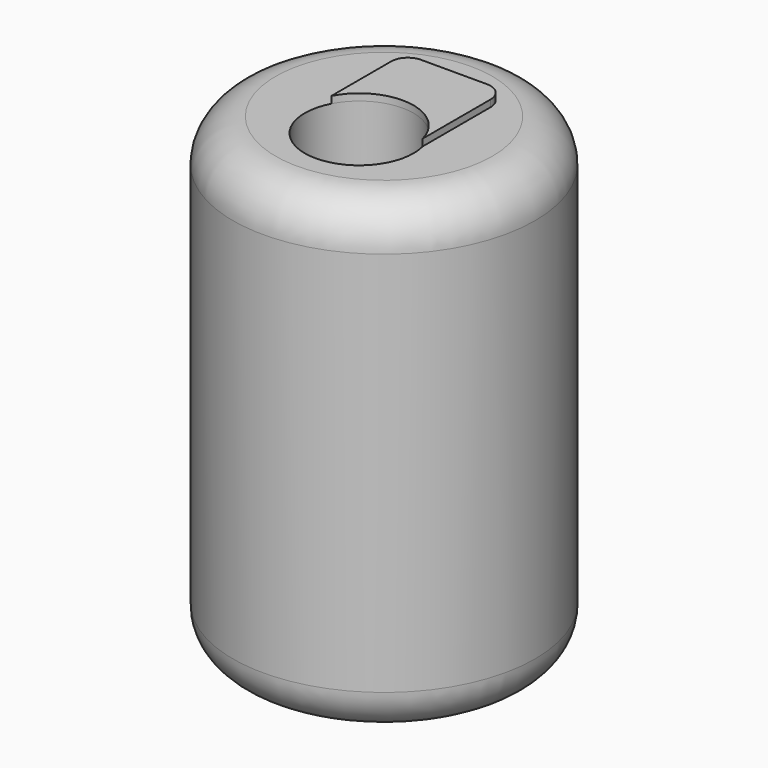
from build123d import *

# Parameters (mm, degrees)
F0_R     = 17.6630626633
F1_DEPTH = 55.1
F2_R     = 5
F3_R     = 6.360255015
F4_DEPTH = 4.4
F5_DEPTH = 9.1
F6_DEPTH = 6.2
F8_DEPTH = 0.8
F9_R     = 2.1727922061
F10_R    = 1.9313708499


# Not quite as in the source:
# - the program builds the solid bodies; features that only make, move or delete a surface that nothing else refers to are left out


with BuildPart() as f1:
    # F0 (on Top) → F1 (new body)
    with BuildSketch(Plane.XY):
        with Locations((-60.169108212, 0)):
            Circle(F0_R)
    extrude(amount=F1_DEPTH)

    # F2
    f2_edges = [f1.edges().sort_by_distance(p)[0] for p in [
        (-77.832171, 0, 0),
        (-77.832171, 0, 55.1),
    ]]
    fillet(f2_edges, radius=F2_R)

    # F3 (on face) → F4 (join)
    with BuildSketch(Plane.XY.offset(55.1)):
        with Locations((-59.8526485264, -4.0257023647)):
            Circle(F3_R)
    extrude(amount=F4_DEPTH)

    # F5 (cut): a face of the model
    f5_faces = [f1.faces().sort_by_distance(p)[0] for p in [
        (-59.8526485264, -4.0257023647, 59.5),
    ]]
    extrude(f5_faces, amount=-F5_DEPTH, mode=Mode.SUBTRACT)

    # F6 (cut): a face of the model
    f6_faces = [f1.faces().sort_by_distance(p)[0] for p in [
        (-59.8526485264, -4.0257023647, 50.4),
    ]]
    extrude(f6_faces, amount=-F6_DEPTH, mode=Mode.SUBTRACT)

    # F7 (on face) → F8 (join)
    with BuildSketch(Plane.XY.offset(55.1)):
        with BuildLine():
            Line((-53.6922231234, 9.6299564466), (-65.4776543379, 9.6299564466))
            Line((-65.4776543379, 9.6299564466), (-65.4776543379, -1.0571752086))
            ThreePointArc((-65.4776543379, -1.0571752086), (-59.1093847847, 2.2909742033), (-53.6922231234, -2.4439303493))
            Line((-53.6922231234, -2.4439303493), (-53.6922231234, 9.6299564466))
        make_face()
    extrude(amount=F8_DEPTH)

    # F9
    f9_edges = [f1.edges().sort_by_distance(p)[0] for p in [
        (-53.692223, 9.629956, 55.5),
    ]]
    fillet(f9_edges, radius=F9_R)

    # F10
    f10_edges = [f1.edges().sort_by_distance(p)[0] for p in [
        (-65.477654, 9.629956, 55.5),
    ]]
    fillet(f10_edges, radius=F10_R)


solid = f1.part
